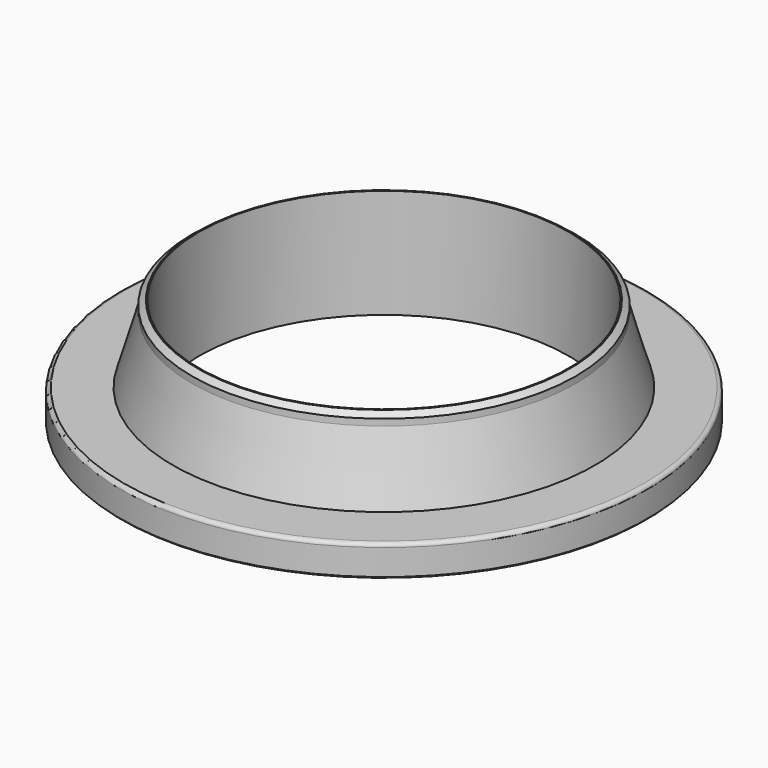
from build123d import *

# Parameters (mm, degrees)
F2_R    = 5
F3_SIZE = 2


with BuildPart() as f1:
    # F0 (on Front) → F1 (revolve)
    with BuildSketch(Plane.XZ):
        Polygon((-79.4498865843, -12.1671419008), (-79.4498865843, 132.3328580992), (-81.0498865843, 132.3328580992), (-88.9998865843, 126.2326085448), (-88.9998865843, 117.5993978977), (-114.3998865843, 30.7328580992), (-184.2498865843, 30.7328580992), (-184.2498865843, -10.5671419008), (-127.0998865843, -10.5671419008), (-127.0998865843, -12.1671419008), align=None)
    revolve(axis=Axis((165.0001134157, 0, 0.9622275829), (0, 0, -1)))

    # F2
    f2_edges = [f1.edges().sort_by_distance(p)[0] for p in [
        (514.250113, 0, 30.732858),
    ]]
    fillet(f2_edges, radius=F2_R)

    # F3
    f3_edges = [f1.edges().sort_by_distance(p)[0] for p in [
        (514.250113, 0, -10.567142),
    ]]
    chamfer(f3_edges, length=F3_SIZE)


solid = f1.part
